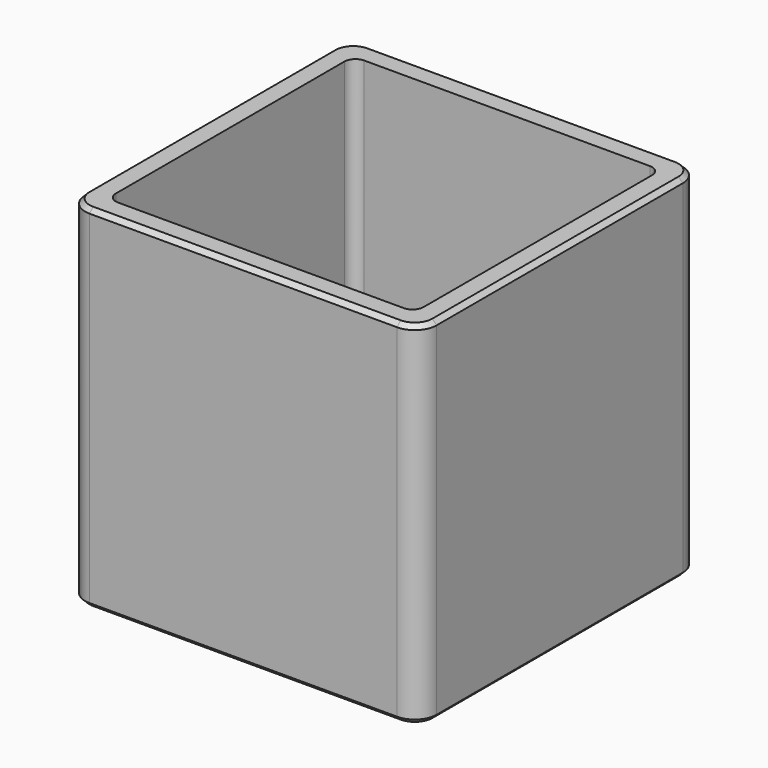
from build123d import *

# Parameters (mm, degrees)
F1_DEPTH = 80
F2_T     = 5
F3_R     = 2.5
F4_SIZE  = 1


# Not quite as in the source:
# - a shell that OpenCascade refuses in one call is made with other operations: the cavity is built on its own and cut out


with BuildPart() as f1:
    # F0 (on Top) → F1 (new body)
    with BuildSketch(Plane.XY):
        with BuildLine():
            Line((35, 40), (-35, 40))
            ThreePointArc((-35, 40), (-38.5355339059, 38.5355339059), (-40, 35))
            Line((-40, 35), (-40, -35))
            ThreePointArc((-40, -35), (-38.5355339059, -38.5355339059), (-35, -40))
            Line((-35, -40), (35, -40))
            ThreePointArc((35, -40), (38.5355339059, -38.5355339059), (40, -35))
            Line((40, -35), (40, 35))
            ThreePointArc((40, 35), (38.5355339059, 38.5355339059), (35, 40))
        make_face()
    extrude(amount=F1_DEPTH)

    # F2: shell of thickness 5, made by hand


with BuildPart() as f2_core1:
    # F2_t2: copy of F1
    add(f1.part)

    # the walls: a layer under each face that stays
    f2_faces = [f2_core1.faces().sort_by_distance(p)[0] for p in [
        (0, 40, 40),
        (-40, 0, 40),
        (0, -40, 40),
        (40, 0, 40),
        (0, 0, 0),
    ]]
    thicken(f2_faces, amount=-F2_T, mode=Mode.SUBTRACT)


with BuildPart() as f1_1:
    add(f1.part)

    # what is left inside the walls is the cavity
    f2_cavity = [f2_core1.part.solids().sort_by_distance(p)[0] for p in [
        (0, 34.95, 55),
    ]]
    add(f2_cavity, mode=Mode.SUBTRACT)

    # F3
    f3_edges = [f1_1.edges().sort_by_distance(p)[0] for p in [
        (35, 35, 42.5),
        (-35, 35, 42.5),
        (-35, -35, 42.5),
        (35, -35, 42.5),
        (35, 0, 5),
        (0, -35, 5),
        (-35, 0, 5),
        (0, 35, 5),
    ]]
    fillet(f3_edges, radius=F3_R)

    # F4
    f4_edges = [f1_1.edges().sort_by_distance(p)[0] for p in [
        (0, 40, 0),
        (-38.535534, 38.535534, 0),
        (-40, 0, 0),
        (-38.535534, -38.535534, 0),
        (0, -40, 0),
        (38.535534, -38.535534, 0),
        (40, 0, 0),
        (38.535534, 38.535534, 0),
        (0, 40, 80),
        (-38.535534, 38.535534, 80),
    ]]
    chamfer(f4_edges, length=F4_SIZE)


solid = f1_1.part
